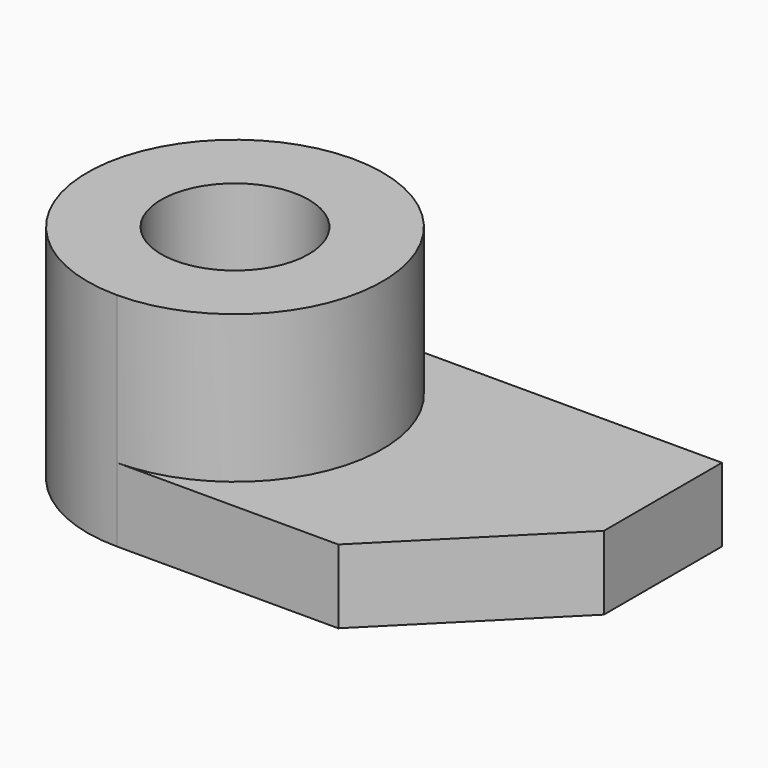
from build123d import *
from build123d import SkipClean  # not in build123d's __all__

# Parameters (mm, degrees)
F1_DEPTH = 19.05
F3_DEPTH = 25.4
F4_R     = 6.35
F5_DEPTH = 25.4
F7_DEPTH = 12.7


with BuildPart() as f1:
    # F0 (on Top) → F1 (new body)
    with BuildSketch(Plane.XY):
        with BuildLine():
            ThreePointArc((0, -12.7), (8.9802561211, -8.9802561211), (12.7, 0))
            ThreePointArc((12.7, 0), (8.9802561211, 8.9802561211), (0, 12.7))
            ThreePointArc((0, 12.7), (-12.7, 0), (0, -12.7))
        make_face()
        with BuildLine():
            ThreePointArc((0, 12.7), (8.9802561211, 8.9802561211), (12.7, 0))
            ThreePointArc((12.7, 0), (8.9802561211, -8.9802561211), (0, -12.7))
            Line((0, -12.7), (31.75, -12.7))
            Line((31.75, -12.7), (31.75, 12.7))
            Line((31.75, 12.7), (0, 12.7))
        make_face()
    extrude(amount=-F1_DEPTH)

    # F2 (on Top) → F3 (cut)
    with BuildSketch(Plane.XY):
        Polygon((31.75, 0), (19.05, -12.7), (31.75, -12.7), align=None)
    extrude(amount=-F3_DEPTH, mode=Mode.SUBTRACT)

    # F4 (on Top) → F5 (cut)
    with BuildSketch(Plane.XY):
        Circle(F4_R)
    extrude(amount=-F5_DEPTH, mode=Mode.SUBTRACT)

    # F6 (on Top) → F7 (cut)
    with BuildSketch(Plane.XY):
        with BuildLine():
            Line((36.2295210361, 12.7), (0, 12.7))
            ThreePointArc((0, 12.7), (12.7, 0), (0, -12.7))
            Line((0, -12.7), (36.2295210361, -12.7))
            Line((36.2295210361, -12.7), (36.2295210361, 12.7))
        make_face()
    with SkipClean():  # cleaning this boolean's faces spoils the solid; the shape is the same uncleaned
        extrude(amount=-F7_DEPTH, mode=Mode.SUBTRACT)


solid = f1.part
